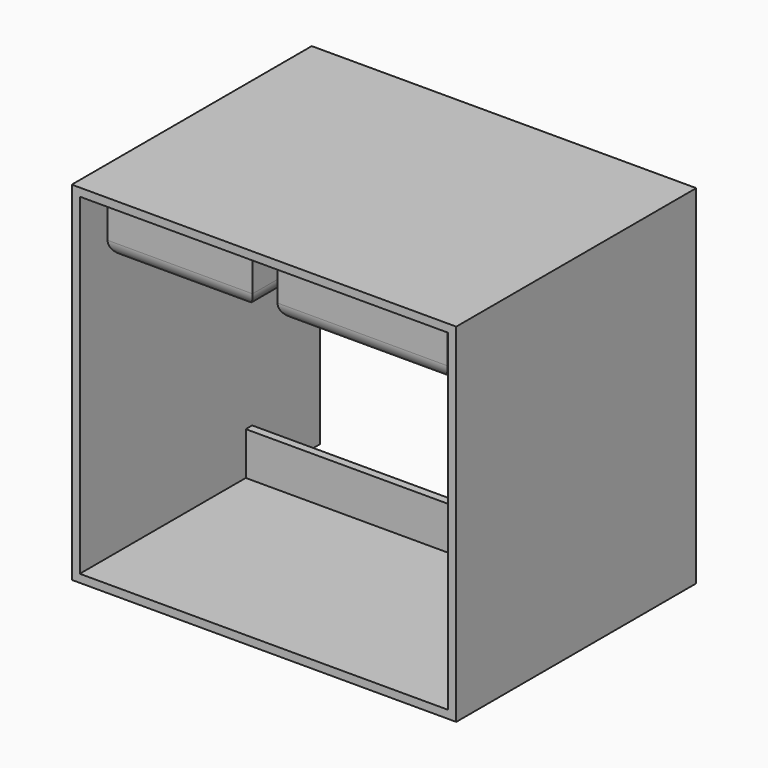
from build123d import *

# Parameters (mm, degrees)
F0_W      = 769
F0_H      = 696
F0_W_2    = 737
F0_H_2    = 664
F1_DEPTH  = 600
F2_W      = 737
F2_H      = 16
F3_DEPTH  = 86
F4_W      = 290
F4_H      = 400
F4_W_2    = 340
F5_DEPTH  = 110
F6_R      = 30
F7_W      = 737
F7_H      = 169
F8_DEPTH  = 16
F9_R      = 25
F10_DEPTH = 40
F11_R     = 25
F12_DEPTH = 40
F13_R     = 15
F14_ANGLE = 40


# Not quite as in the source:
# - a feature of the source that left no trace in its solid (it failed there, or was rolled back) is left out
# - a pattern or mirror of a feature is missing from the dataset's text; its kind, count and spacing are read off the source's solid


with BuildPart() as f1:
    # F0 (on Front) → F1 (new body)
    with BuildSketch(Plane.XZ):
        with Locations((368.5, 332)):
            Rectangle(F0_W, F0_H)
        with Locations((368.5, 332)):
            Rectangle(F0_W_2, F0_H_2, mode=Mode.SUBTRACT)
    extrude(amount=-F1_DEPTH)

    # F2 (on face) → F3 (join)
    with BuildSketch(Plane.XY):
        with Locations((368.5, 423)):
            Rectangle(F2_W, F2_H)
    extrude(amount=F3_DEPTH)

    # F4 (on face) → F5 (join)
    with BuildSketch(Plane(origin=(0, 0, 664), x_dir=(1, 0, 0), z_dir=(0, 0, -1))):
        with Locations((175, -232)):
            Rectangle(F4_W, F4_H)
        with Locations((540, -232)):
            Rectangle(F4_W_2, F4_H)
    extrude(amount=F5_DEPTH)

    # F6
    f6_edges = [f1.edges().sort_by_distance(p)[0] for p in [
        (175, 32, 554),
        (30, 232, 554),
        (175, 432, 554),
        (320, 232, 554),
        (540, 32, 554),
        (370, 232, 554),
        (540, 432, 554),
        (710, 232, 554),
    ]]
    fillet(f6_edges, radius=F6_R)

    # F7 (on face) → F8 (cut, through all)
    with BuildSketch(Plane.XY):
        with Locations((368.5, 515.5)):
            Rectangle(F7_W, F7_H)
    extrude(amount=-F8_DEPTH, mode=Mode.SUBTRACT)

    # F9 (on face) → F10 (join)
    with BuildSketch(Plane(origin=(0, 0, 554), x_dir=(1, 0, 0), z_dir=(0, 0, -1))):
        with Locations((175, -367)):
            Circle(F9_R)
    extrude(amount=F10_DEPTH)

    # F11 (on face) → F12 (join)
    with BuildSketch(Plane(origin=(0, 0, 554), x_dir=(1, 0, 0), z_dir=(0, 0, -1))):
        with Locations((450, -367)):
            Circle(F11_R)
    extrude(amount=F12_DEPTH)

    # F13 (on face) → F14 (revolve)
    with BuildSketch(Plane(origin=(0, 0, 514), x_dir=(1, 0, 0), z_dir=(0, 0, -1))):
        with Locations((450, -367)):
            Circle(F13_R)
    f14 = revolve(axis=Axis((540, 402, 554), (1, 0, 0)), revolution_arc=F14_ANGLE)

    # F14_copies: F14 across plane
    add(f14.mirror(Plane(origin=(312.5, 0, 0), x_dir=(0, 0, -1), z_dir=(-1, 0, 0))))


solid = f1.part
